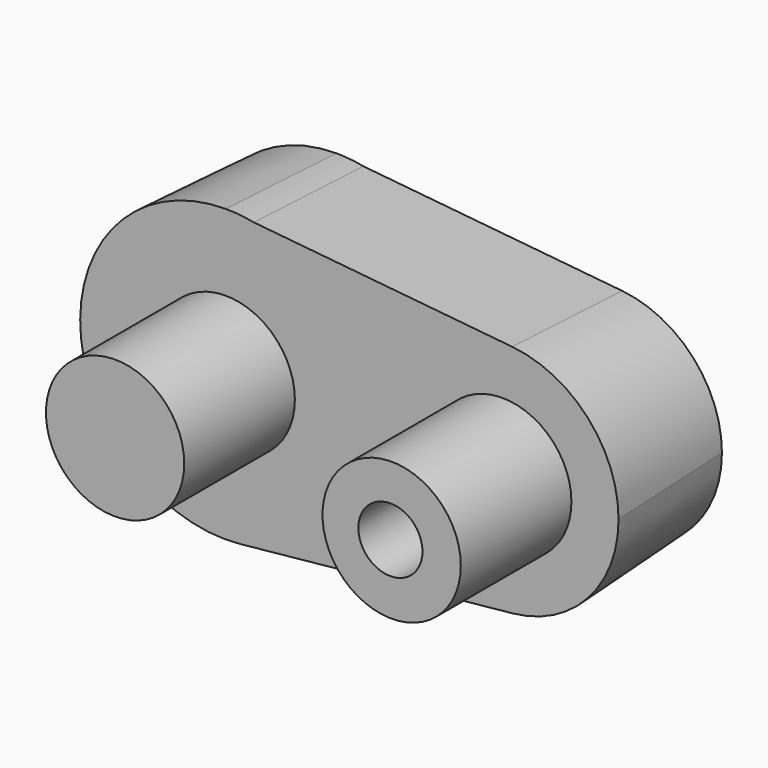
from build123d import *

# Parameters (mm, degrees)
F1_DEPTH = 25
F1_TAPER = -3
F2_R     = 12.5
F3_DEPTH = 50
F4_R     = 5.7994178108
F5_DEPTH = 50
F7_DEPTH = 10


# Not quite as in the source:
# - a feature names something its author has since deleted; it is built from what else it names


with BuildPart() as f1:
    # F0 (on Front) → F1 (new body)
    with BuildSketch(Plane.XZ):
        with BuildLine():
            Line((4.8843180895, 24.5182266243), (0, 25))
            ThreePointArc((0, 25), (-24.9682800601, -1.2589641933), (2.5147336452, -24.8732007328))
            ThreePointArc((2.5147336452, -24.8732007328), (18.5454622635, -16.7650180267), (25, 0))
            ThreePointArc((25, 0), (19.3275444927, 15.8570496588), (4.8843180895, 24.5182266243))
        make_face()
        with BuildLine():
            ThreePointArc((4.8843180895, 24.5182266243), (2.4540104311, 24.8792651178), (0, 25))
            Line((0, 25), (4.8843180895, 24.5182266243))
        make_face()
        with BuildLine():
            ThreePointArc((25, 0), (18.5454622635, -16.7650180267), (2.5147336452, -24.8732007328))
            Line((2.5147336452, -24.8732007328), (51.7188404795, -19.8985605862))
            ThreePointArc((51.7188404795, -19.8985605862), (29.7070684597, -0.0244101143), (51.6702619082, 19.9034120943))
            Line((51.6702619082, 19.9034120943), (4.8843180895, 24.5182266243))
            ThreePointArc((4.8843180895, 24.5182266243), (19.3275444927, 15.8570496588), (25, 0))
        make_face()
        with BuildLine():
            ThreePointArc((51.6702619082, 19.9034120943), (29.7070684597, -0.0244101143), (51.7188404795, -19.8985605862))
            ThreePointArc((51.7188404795, -19.8985605862), (64.5434233741, -13.4120144213), (69.7070535633, 0))
            ThreePointArc((69.7070535633, 0), (64.5270428835, 13.430112306), (51.6702619082, 19.9034120943))
        make_face()
    extrude(amount=F1_DEPTH, taper=F1_TAPER)

    # F2 (on Front) → F3 (join)
    with BuildSketch(Plane.XZ):
        Circle(F2_R)
        with Locations((50, 0)):
            Circle(F2_R)
    extrude(amount=F3_DEPTH)

    # F4 (on Front) → F5 (cut)
    with BuildSketch(Plane.XZ):
        with Locations((49.772053957, 0)):
            Circle(F4_R)
    extrude(amount=F5_DEPTH, mode=Mode.SUBTRACT)

    # F6 (on Front) → F7 (join)
    with BuildSketch(Plane.XZ):
        Polygon((-0.0836669881, -5.4505592747), (4.6784893026, -2.7977373745), (4.7621562908, 2.6528219002), (0.0836669881, 5.4505592747), (-4.6784893026, 2.7977373745), (-4.7621562908, -2.6528219002), align=None)
    extrude(amount=-F7_DEPTH)


solid = f1.part
